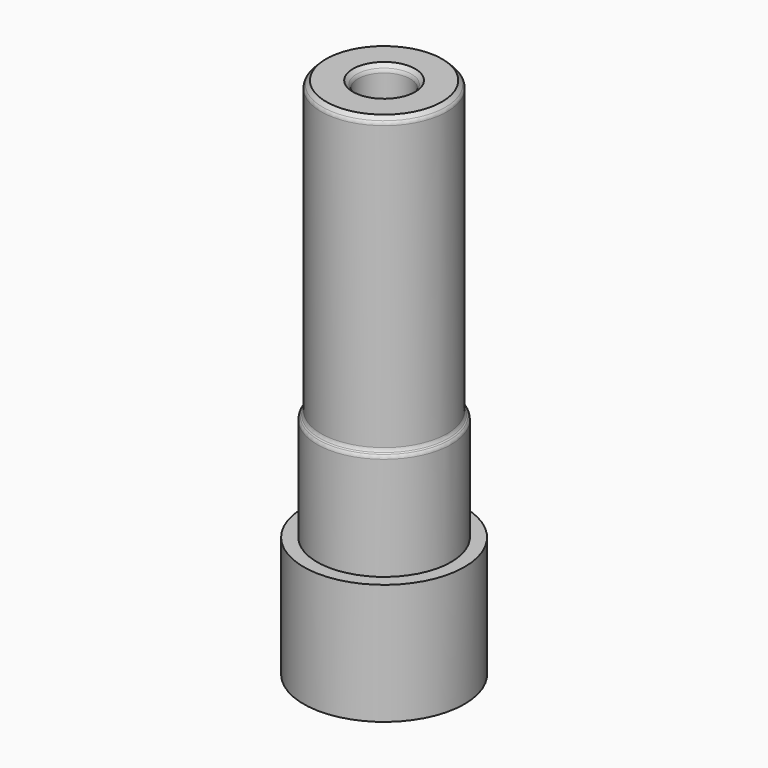
from build123d import *

# Parameters (mm, degrees)
F0_R        = 6.665
F0_R_2      = 6.265
F1_DEPTH    = 11
F2_DEPTH    = 40
F0_R_3      = 8
F3_DEPTH    = 12
F4_R        = 2.6
F5_DEPTH    = 52
F6_S5_R     = 6.265
F6_T6_DEPTH = 11
F7_R        = 0.5
F8_R        = 0.5


# Not quite as in the source:
# - a fillet or chamfer that OpenCascade refuses, or shapes differently, is made with other operations: its cross-section is extruded or revolved along the edge and cut away or added


with BuildPart() as f1:
    # F0 (on Top) → F1 (new body)
    with BuildSketch(Plane.XY):
        Circle(F0_R)
        Circle(F0_R_2, mode=Mode.SUBTRACT)
        Circle(F0_R_2)
    extrude(amount=F1_DEPTH)

    # F0 (on Top) → F2 (join)
    with BuildSketch(Plane.XY):
        Circle(F0_R_2)
    extrude(amount=F2_DEPTH)

    # F0 (on Top) → F3 (join)
    with BuildSketch(Plane.XY):
        Circle(F0_R_3)
        Circle(F0_R, mode=Mode.SUBTRACT)
        Circle(F0_R)
        Circle(F0_R_2, mode=Mode.SUBTRACT)
        Circle(F0_R_2)
    extrude(amount=-F3_DEPTH)

    # F4 (on face) → F5 (cut)
    with BuildSketch(Plane(origin=(0, 0, -12), x_dir=(1, 0, 0), z_dir=(0, 0, -1))):
        Circle(F4_R)
    extrude(amount=-F5_DEPTH, mode=Mode.SUBTRACT)

    # F6: chamfer of 0.5 on 4 edges, made by hand


with BuildPart() as f6_tool2:
    # F6_s3 → F6_t4 (revolve)
    with BuildSketch(Plane.XZ):
        Polygon((6.665, 10.5), (6.165, 11), (6.665, 11), align=None)
    revolve(axis=Axis((0, 0, 11), (0, 0, 1)))

    # F6_s5 → F6_t6 (cut, symmetric)
    with BuildSketch(Plane.XY.offset(10.8)):
        Circle(F6_S5_R)
    extrude(amount=F6_T6_DEPTH, both=True, mode=Mode.SUBTRACT)


with BuildPart() as f1_1:
    add(f1.part)

    # F6_t1: cut F6_tool2
    add(f6_tool2.part, mode=Mode.SUBTRACT)

    # F6_s7 → F6_t8 (revolve, cut)
    with BuildSketch(Plane.XZ):
        Polygon((5.765, 40), (6.265, 39.5), (6.265, 40), align=None)
    revolve(axis=Axis((0, 0, 40), (0, 0, 1)), mode=Mode.SUBTRACT)

    # F6_s9 → F6_t10 (revolve, cut)
    with BuildSketch(Plane.XZ):
        Polygon((2.6, 39.5), (3.1, 40), (2.6, 40), align=None)
    revolve(axis=Axis((0, 0, 40), (0, 0, -1)), mode=Mode.SUBTRACT)

    # F6_s11 → F6_t12 (revolve, cut)
    with BuildSketch(Plane.XZ):
        Polygon((3.1, -12), (2.6, -11.5), (2.6, -12), align=None)
    revolve(axis=Axis((0, 0, -12), (0, 0, -1)), mode=Mode.SUBTRACT)

    # F7
    f7_edges = [f1_1.edges().sort_by_distance(p)[0] for p in [
        (-6.665, 0, 10.5),
        (-6.265, 0, 39.5),
        (-2.6, 0, 39.5),
        (-2.6, 0, -11.5),
    ]]
    fillet(f7_edges, radius=F7_R)

    # F8
    f8_edges = [f1_1.edges().sort_by_distance(p)[0] for p in [
        (-6.265, 0, 10.9),
    ]]
    fillet(f8_edges, radius=F8_R)


solid = f1_1.part
